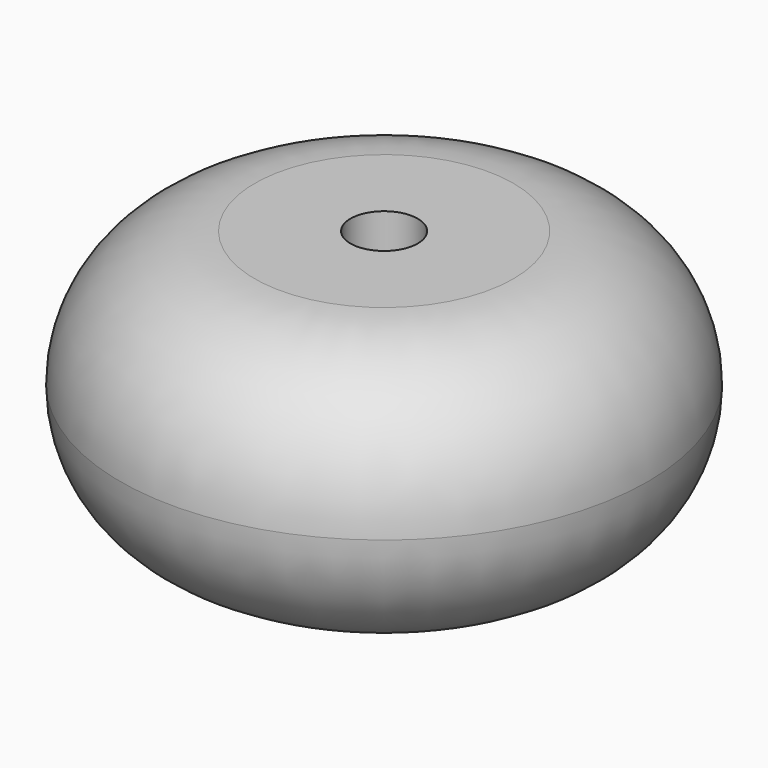
from build123d import *

# Parameters (mm, degrees)
F0_R     = 24.9021942903
F1_DEPTH = 25.4
F2_R     = 12.69999
F3_R     = 3.175
F4_DEPTH = 25.401


# Not quite as in the source:
# - a fillet or chamfer is up to 0.001 mm smaller than in the source, because OpenCascade refuses the exact size


with BuildPart() as f1:
    # F0 (on Top) → F1 (new body)
    with BuildSketch(Plane.XY):
        Circle(F0_R)
    extrude(amount=F1_DEPTH)

    # F2 (radius 12.7 in the source; OpenCascade refuses exactly that, so slightly less here)
    f2_edges = [f1.edges().sort_by_distance(p)[0] for p in [
        (-24.902194, 0, 0),
        (-24.902194, 0, 25.4),
    ]]
    fillet(f2_edges, radius=F2_R)

    # F3 (on face) → F4 (cut, through all)
    with BuildSketch(Plane.XY.offset(25.4)):
        Circle(F3_R)
    extrude(amount=-F4_DEPTH, mode=Mode.SUBTRACT)


solid = f1.part
